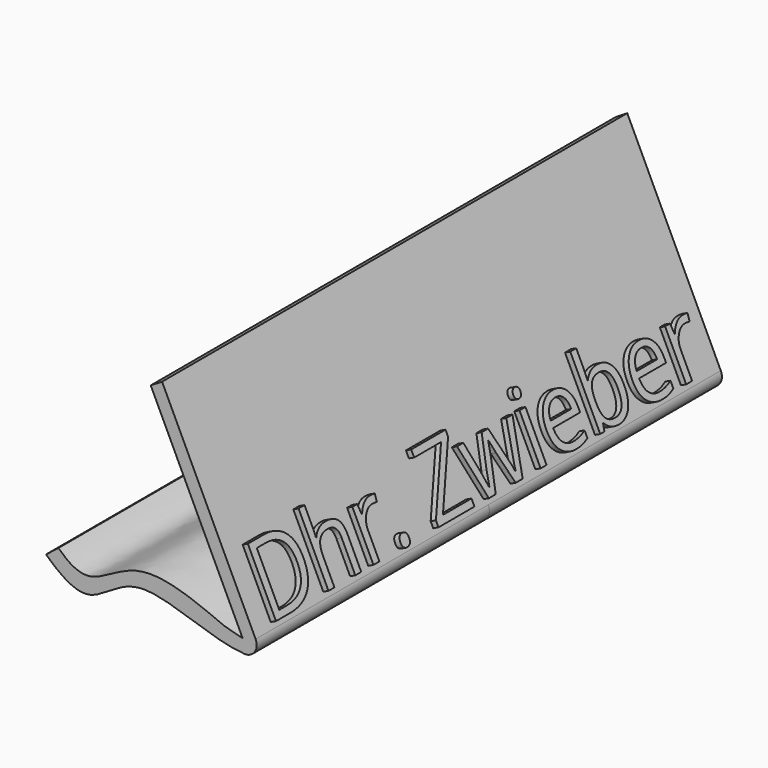
from build123d import *

# Parameters (mm, degrees)
F1_DEPTH      = 100
F1_DEPTH_BACK = 100
F2_R          = 4
F3_TEXT_SIZE  = 31.4828202439
F4_DEPTH      = 2


# Not quite as in the source:
# - Text() gives the source's letters only with a copy of the font that has no kerning and outlines rounded to 1/6400 em; it was checked with that copy


with BuildPart() as f1:
    # F0 (on Front) → F1 (new body, two sides)
    with BuildSketch(Plane.XZ) as f1_sk:
        with BuildLine():
            Line((33.3748926994, -27.0979408562), (0, 42.9020591438))
            Line((0, 42.9020591438), (-3.9007712825, 40.5167356237))
            Line((-3.9007712825, 40.5167356237), (27.7016319892, -25.7656716018))
            add(Edge.make_bspline(
                [(27.7016319892, -25.7656716018), (29.2316382, -26.1352362057), (31.0840432446, -26.5690450229), (33.3748926994, -27.0979408562)],
                knots=[0.9521623536, 0.9521623536, 0.9521623536, 0.9521623536, 1, 1, 1, 1], degree=3))
        make_face()
        with BuildLine():
            Line((34.6386361346, -29.7484974066), (33.3748926994, -27.0979408562))
            add(Edge.make_bspline(
                [(27.7016319892, -25.7656716018), (29.2316382, -26.1352362057), (31.0840432446, -26.5690450229), (33.3748926994, -27.0979408562)],
                knots=[0.9521623536, 0.9521623536, 0.9521623536, 0.9521623536, 1, 1, 1, 1], degree=3))
            add(Edge.make_bspline(
                [(-35.6504382531, -19.0559427176), (-32.0179856242, -22.5451874705), (-24.0718451477, -27.4567719869), (-7.9249887862, -11.7429865299), (19.2399803553, -23.1569476166), (21.4853133253, -24.2641539424), (27.7016319892, -25.7656716018)],
                knots=[0, 0, 0, 0, 0.2056964386, 0.4641948954, 0.7578010155, 0.9521623536, 0.9521623536, 0.9521623536, 0.9521623536], degree=3))
            add(Edge.make_bspline(
                [(-35.6504382531, -19.0559427176), (-36.8797642233, -19.9574482637), (-38.6636613559, -21.4725503747), (-39.8929873261, -22.3740559208)],
                knots=[0, 0, 0, 0, 5.3860094565, 5.3860094565, 5.3860094565, 5.3860094565], degree=3))
            add(Edge.make_bspline(
                [(34.6386361346, -29.7484974066), (22.1278600221, -33.0702515847), (-8.0878186624, -13.3017915911), (-24.4067474709, -34.5954696375), (-35.1082672403, -26.8971077222), (-39.8929873261, -22.3740559208)],
                knots=[0, 0, 0, 0, 0.4363542022, 0.7294414987, 1, 1, 1, 1], degree=3))
        make_face()
    extrude(amount=F1_DEPTH)
    extrude(f1_sk.sketch, amount=-F1_DEPTH_BACK)

    # F2
    f2_edges = [f1.edges().sort_by_distance(p)[0] for p in [
        (34.638636, 50, -29.748497),
        (34.638636, -50, -29.748497),
    ]]
    fillet(f2_edges, radius=F2_R)

    # F3 (on face) → F4 (join)
    with BuildSketch(Plane(origin=(16.6663710824, 0, 7.9462620938), x_dir=(0, 1, 0), z_dir=(0.9026523891, 0, 0.4303703805))):
        with Locations((-95.5, -34.0374756127)):
            Text('Dhr. Zwieber', F3_TEXT_SIZE, font='Open Sans', text_align=(TextAlign.LEFT, TextAlign.BOTTOM))
    extrude(amount=F4_DEPTH)


solid = f1.part
